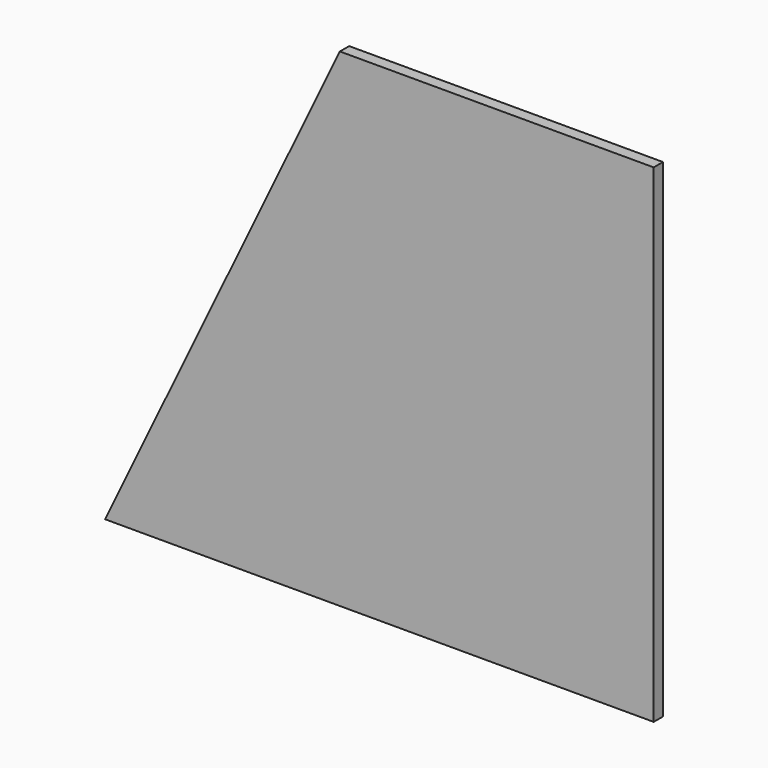
from build123d import *

# Parameters (mm, degrees)
F0_W        = 165.1
F0_H        = 133.35
F1_DEPTH    = 1.5875
F2_T1_DEPTH = 858.0326548283


# Not quite as in the source:
# - a fillet or chamfer that OpenCascade refuses, or shapes differently, is made with other operations: its cross-section is extruded or revolved along the edge and cut away or added


with BuildPart() as f1:
    # F0 (on Front) → F1 (new body, symmetric)
    with BuildSketch(Plane.XZ):
        Rectangle(F0_W, F0_H)
    extrude(amount=F1_DEPTH, both=True)

    # F2: chamfer of 165 x 79.375 on 1 edges, made by hand

    # F2_s2 → F2_t1 (cut)
    with BuildSketch(Plane.XZ.offset(-429.0163274141)):
        Polygon((-82.55, -98.325), (-3.175, 66.675), (-82.55, 66.675), align=None)
    extrude(amount=F2_T1_DEPTH, mode=Mode.SUBTRACT)


solid = f1.part
